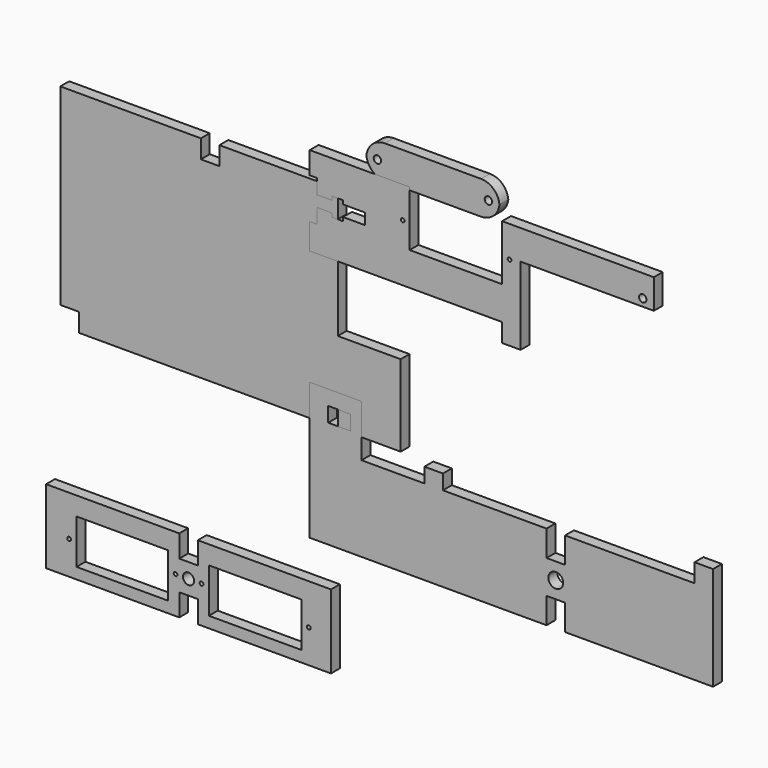
from build123d import *

# Parameters (mm, degrees)
F1_DEPTH    = 3
F2_R        = 2
F2_W        = 6
F2_H        = 4
F3_DEPTH    = 3
F4_R        = 0.5
F4_W        = 24.7760626674
F4_H        = 12
F4_R_2      = 1.5
F4_W_2      = 25
F5_DEPTH    = 3
F6_W        = 36
F6_H        = 9
F6_R        = 1
F7_DEPTH    = 3
F8_T1_DEPTH = 28
F9_R        = 0.5
F9_R_2      = 1
F10_DEPTH   = 3


# Not quite as in the source:
# - a fillet or chamfer that OpenCascade refuses, or shapes differently, is made with other operations: its cross-section is extruded or revolved along the edge and cut away or added


with BuildPart() as f1:
    # F0 (on Front) → F1 (new body)
    with BuildSketch(Plane.XZ):
        Polygon((-29.4190670252, 48.4748313129), (-67.4190670252, 48.4748313129), (-67.4190670252, -3.5251686871), (-62.4190670252, -3.5251686871), (-62.4190670252, -8.5251686871), (2.5809329748, -8.5251686871), (2.5809329748, -3.5251686871), (7.5809329748, -3.5251686871), (7.5809329748, -8.5251686871), (24.5809329748, -8.5251686871), (24.5809329748, 13.4748313129), (7.5809329748, 13.4748313129), (7.5809329748, 48.4748313129), (-24.4190670252, 48.4748313129), (-24.4190670252, 43.4748313129), (-29.4190670252, 43.4748313129), align=None)
    extrude(amount=F1_DEPTH)


with BuildPart() as f3:
    # F2 (on Front) → F3 (new body)
    with BuildSketch(Plane.XZ):
        Polygon((14, 0), (0, 0), (0, -37), (64, -37), (64, -30), (69, -30), (69, -37), (109, -37), (109, -9), (104, -9), (104, -14), (69, -14), (69, -21), (64, -21), (64, -14), (36, -14), (36, -10), (31, -10), (31, -14), (14, -14), align=None)
        with Locations((66.5, -25.5)):
            Circle(F2_R, mode=Mode.SUBTRACT)
        with Locations((8, -6)):
            Rectangle(F2_W, F2_H, mode=Mode.SUBTRACT)
    extrude(amount=F3_DEPTH)


with BuildPart() as f5:
    # F4 (on Front) → F5 (new body)
    with BuildSketch(Plane.XZ):
        Polygon((-71.2518001199, -47.4190670252), (-71.2518001199, -67.4190670252), (-35.2518001199, -67.4190670252), (-35.2518001199, -61.4190670252), (-30.2518001199, -61.4190670252), (-30.2518001199, -67.4190670252), (5.7481998801, -67.4190670252), (5.7481998801, -47.4190670252), (-30.2518001199, -47.4190670252), (-30.2518001199, -53.4190670252), (-35.2518001199, -53.4190670252), (-35.2518001199, -47.4190670252), align=None)
        with Locations((-65.0278627872, -58.4190629094)):
            Circle(F4_R, mode=Mode.SUBTRACT)
        with Locations((-50.6398314536, -58.4190629094)):
            Rectangle(F4_W, F4_H, mode=Mode.SUBTRACT)
        with Locations((-36.2518001199, -57.4190670252)):
            Circle(F4_R, mode=Mode.SUBTRACT)
        with Locations((-32.7518001199, -57.4190670252)):
            Circle(F4_R_2, mode=Mode.SUBTRACT)
        with Locations((-29.2518001199, -57.4190670252)):
            Circle(F4_R, mode=Mode.SUBTRACT)
        with Locations((-14.7518001199, -58.4190629094)):
            Rectangle(F4_W_2, F4_H, mode=Mode.SUBTRACT)
        with Locations((-0.2518001199, -58.4190629094)):
            Circle(F4_R, mode=Mode.SUBTRACT)
    extrude(amount=F5_DEPTH)


with BuildPart() as f7:
    # F6 (on Front) → F7 (new body)
    with BuildSketch(Plane.XZ):
        with Locations((33.2967646718, 58.9532347322)):
            Rectangle(F6_W, F6_H)
        with Locations((18.2967646718, 58.9532347322)):
            Circle(F6_R, mode=Mode.SUBTRACT)
        with Locations((48.2967646718, 58.9532347322)):
            Circle(F6_R, mode=Mode.SUBTRACT)
    extrude(amount=F7_DEPTH)

    # F8: fillet of radius 5 on 4 edges, made by hand

    # F8_s2 → F8_t1 (cut)
    with BuildSketch(Plane.XZ.offset(-12.5)):
        with BuildLine():
            ThreePointArc((20.2967646718, 63.4532347322), (16.7612307659, 61.9887686381), (15.2967646718, 58.4532347322))
            Line((15.2967646718, 58.4532347322), (15.2967646718, 63.4532347322))
            Line((15.2967646718, 63.4532347322), (20.2967646718, 63.4532347322))
        make_face()
        with BuildLine():
            ThreePointArc((15.2967646718, 59.4532347322), (16.7612307659, 55.9177008262), (20.2967646718, 54.4532347322))
            Line((20.2967646718, 54.4532347322), (15.2967646718, 54.4532347322))
            Line((15.2967646718, 54.4532347322), (15.2967646718, 59.4532347322))
        make_face()
        with BuildLine():
            ThreePointArc((46.2967646718, 63.4532347322), (49.8322985777, 61.9887686381), (51.2967646718, 58.4532347322))
            Line((51.2967646718, 58.4532347322), (51.2967646718, 63.4532347322))
            Line((51.2967646718, 63.4532347322), (46.2967646718, 63.4532347322))
        make_face()
        with BuildLine():
            ThreePointArc((46.2967646718, 54.4532347322), (49.8322985777, 55.9177008262), (51.2967646718, 59.4532347322))
            Line((51.2967646718, 59.4532347322), (51.2967646718, 54.4532347322))
            Line((51.2967646718, 54.4532347322), (46.2967646718, 54.4532347322))
        make_face()
    extrude(amount=F8_T1_DEPTH, mode=Mode.SUBTRACT)


with BuildPart() as f10:
    # F9 (on Front) → F10 (new body)
    with BuildSketch(Plane.XZ):
        Polygon((27, 55.2383102477), (0, 55.2383102477), (0, 49.2383102477), (2, 49.2383102477), (2, 45.2383102477), (6, 45.2383102477), (6, 46.2383102477), (9, 46.2383102477), (9, 45.2383102477), (15, 45.2383102477), (15, 42.2383102477), (9, 42.2383102477), (9, 41.2383102477), (6, 41.2383102477), (6, 42.2383102477), (2, 42.2383102477), (2, 38.2383102477), (0, 38.2383102477), (0, 31.2383102477), (52, 31.2383102477), (52, 26.2383102477), (57, 26.2383102477), (57, 47.2383102477), (93, 47.2383102477), (93, 55.2383102477), (52, 55.2383102477), (52, 40.2383102477), (27, 40.2383102477), align=None)
        with Locations((25.1189991832, 46.7383102477)):
            Circle(F9_R, mode=Mode.SUBTRACT)
        with Locations((53.9999991832, 46.7383102477)):
            Circle(F9_R, mode=Mode.SUBTRACT)
        with Locations((90, 49.2383102477)):
            Circle(F9_R_2, mode=Mode.SUBTRACT)
    extrude(amount=F10_DEPTH)


solid = Compound([f1.part, f3.part, f5.part, f7.part, f10.part])
